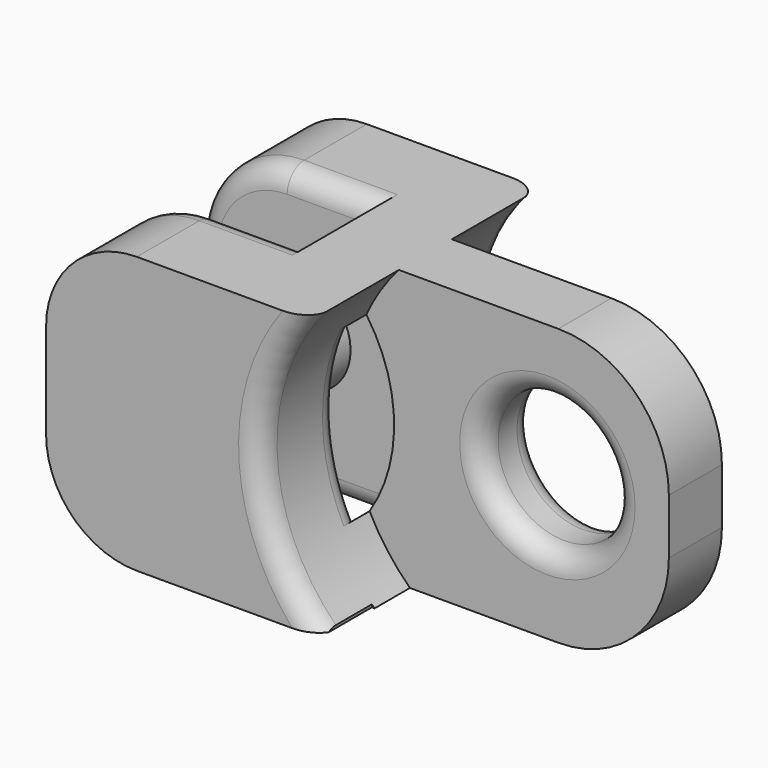
from build123d import *

# Parameters (mm, degrees)
F0_W           = 5
F0_H           = 6
F0_H_2         = 1
F0_W_2         = 13.6665210929
F0_W_3         = 3.0392452702
F0_H_3         = 8
F1_DEPTH       = 25
F2_R           = 6
F3_DEPTH       = 16.6
F4_R           = 14
F5_DEPTH       = 4
F6_R           = 4.5
F7_DEPTH       = 26
F8_R           = 18
F9_DEPTH       = 25
F10_R          = 18
F11_DEPTH      = 25
F12_R          = 10
F13_R          = 8.2083261121
F14_T1_DEPTH   = 8.5833477759
F14_T10_ANGLE  = 81.9823622478
F14_S11_R      = 14
F14_T12_DEPTH  = 16
F14_T16_ANGLE  = 81.9823622478
F14_S17_R      = 14
F14_T18_DEPTH  = 17
F14_T20_ANGLE  = 90
F14_T22_ANGLE  = 90
F14_T24_ANGLE  = 117.7013849945
F14_T26_ANGLE  = 117.7013849945
F14_T30_DEPTH  = 13.2473768354
F14_S31_R      = 14
F14_T32_DEPTH  = 8
F14_T37_DEPTH  = 8.4189497106
F14_S38_R      = 14
F14_T39_DEPTH  = 6
F14_T43_DEPTH  = 8.4189497106
F14_S44_R      = 14
F14_T45_DEPTH  = 6
F14_T49_DEPTH  = 8.4189497106
F14_S50_R      = 14
F14_T51_DEPTH  = 6
F14_T55_DEPTH  = 13.2473768354
F14_S57_R      = 14
F14_T58_DEPTH  = 8
F14_T62_DEPTH  = 8.4189497106
F14_S63_R      = 14
F14_T64_DEPTH  = 6
F14_T66_ANGLE  = 90
F14_T70_DEPTH  = 8.4189497106
F14_S71_R      = 14
F14_T72_DEPTH  = 6
F14_T76_DEPTH  = 8.4189497106
F14_S77_R      = 14
F14_T78_DEPTH  = 6
F14_T82_DEPTH  = 13.2473768354
F14_S84_R      = 14
F14_T85_DEPTH  = 8
F14_T89_DEPTH  = 8.4189497106
F14_S90_R      = 14
F14_T91_DEPTH  = 6
F14_T95_DEPTH  = 13.2473768354
F14_S97_R      = 14
F14_T98_DEPTH  = 8
F14_T102_DEPTH = 8.4189497106
F14_S103_R     = 14
F14_T104_DEPTH = 6
F14_T106_ANGLE = 90


# Not quite as in the source:
# - a fillet or chamfer that OpenCascade refuses, or shapes differently, is made with other operations: its cross-section is extruded or revolved along the edge and cut away or added


with BuildPart() as f1:
    # F0 (on Top) → F1 (new body)
    with BuildSketch(Plane.XY):
        Polygon((-5, 7), (-5, 4), (0, 4), (5, 4), (5, 7), align=None)
        Polygon((-5, -7), (5, -7), (5, -4.4536441088), (5, -4), (0, -4), (-5, -4), align=None)
        with Locations((2.5, 0)):
            Rectangle(F0_W, F0_H)
        with Locations((2.5, -3.5)):
            Rectangle(F0_W, F0_H_2)
        with Locations((2.5, 3.5)):
            Rectangle(F0_W, F0_H_2)
        Polygon((-5, -13), (-5, -7), (-5, -4), (-5, 4), (-5, 7), (-5, 13), (-29.6665210929, 13), (-29.6665210929, 4), (-13.0392452702, 4), (-10, 4), (-10, -4), (-13.0392452702, -4), (-29.6665210929, -4), (-29.6665210929, -13), align=None)
        Polygon((-5, 4), (-5, -4), (0, -4), (0, -3), (0, 3), (0, 4), align=None)
        with Locations((11.8332605464, 0)):
            Rectangle(F0_W_2, F0_H)
        with Locations((-11.5196226351, 0)):
            Rectangle(F0_W_3, F0_H_3)
    extrude(amount=F1_DEPTH)

    # F2 (on face) → F3 (cut, symmetric)
    with BuildSketch(Plane.XZ.offset(3)):
        with Locations((7.6787601748, 13.0187581394)):
            Circle(F2_R)
    extrude(amount=F3_DEPTH, both=True, mode=Mode.SUBTRACT)

    # F4 (on Front) → F5 (cut, symmetric)
    with BuildSketch(Plane.XZ):
        with Locations((-20.1836787164, 12.4924527481)):
            Circle(F4_R)
    extrude(amount=F5_DEPTH, both=True, mode=Mode.SUBTRACT)

    # F6 (on face) → F7 (join, through all)
    with BuildSketch(Plane(origin=(0, 13, 0), x_dir=(-1, 0, 0), z_dir=(0, 1, 0))):
        with Locations((20.2261688847, 12.5)):
            Circle(F6_R)
    extrude(amount=-F7_DEPTH)

    # F8 (on face) → F9 (cut)
    with BuildSketch(Plane.XZ.offset(3)):
        with Locations((7.6787601748, 13.0187581394)):
            Circle(F8_R)
        with BuildLine():
            Line((18.6665210929, 0), (5, 0))
            Line((5, 0), (5, 7.6499366742))
            ThreePointArc((5, 7.6499366742), (10.8352961679, 7.9161822679), (13.6787601748, 13.0187581394))
            ThreePointArc((13.6787601748, 13.0187581394), (10.8352961679, 18.1213340109), (5, 18.3875796047))
            Line((5, 18.3875796047), (5, 25))
            Line((5, 25), (18.6665210929, 25))
            Line((18.6665210929, 25), (18.6665210929, 0))
        make_face(mode=Mode.SUBTRACT)
    extrude(amount=F9_DEPTH, mode=Mode.SUBTRACT)

    # F10 (on face) → F11 (cut)
    with BuildSketch(Plane(origin=(0, 3, 0), x_dir=(-1, 0, 0), z_dir=(0, 1, 0))):
        with Locations((-7.6787601748, 13.0187581394)):
            Circle(F10_R)
        with BuildLine():
            Line((-5, 0), (-18.6665210929, 0))
            Line((-18.6665210929, 0), (-18.6665210929, 25))
            Line((-18.6665210929, 25), (-5, 25))
            Line((-5, 25), (-5, 18.3875796047))
            ThreePointArc((-5, 18.3875796047), (-10.8352961679, 18.1213340109), (-13.6787601748, 13.0187581394))
            ThreePointArc((-13.6787601748, 13.0187581394), (-10.8352961679, 7.9161822679), (-5, 7.6499366742))
            Line((-5, 7.6499366742), (-5, 0))
        make_face(mode=Mode.SUBTRACT)
    extrude(amount=F11_DEPTH, mode=Mode.SUBTRACT)

    # F12
    f12_edges = [f1.edges().sort_by_distance(p)[0] for p in [
        (18.666521, 0, 0),
        (18.666521, 0, 25),
    ]]
    fillet(f12_edges, radius=F12_R)

    # F13
    f13_edges = [f1.edges().sort_by_distance(p)[0] for p in [
        (-29.666521, -8.5, 0),
        (-29.666521, 8.5, 0),
        (-29.666521, 8.5, 25),
        (-29.666521, -8.5, 25),
    ]]
    fillet(f13_edges, radius=F13_R)

    # F14: fillet of radius 1.9313708499 on 16 edges, made by hand

    # F14_s2 → F14_t1 (cut)
    with BuildSketch(Plane.XY.offset(8.2083261121)):
        with BuildLine():
            ThreePointArc((-27.735150243, -4), (-29.1008356679, -4.5656854249), (-29.6665210929, -5.9313708499))
            Line((-29.6665210929, -5.9313708499), (-29.6665210929, -4))
            Line((-29.6665210929, -4), (-27.735150243, -4))
        make_face()
        with BuildLine():
            ThreePointArc((-27.735150243, 4), (-29.1008356679, 4.5656854249), (-29.6665210929, 5.9313708499))
            Line((-29.6665210929, 5.9313708499), (-29.6665210929, 4))
            Line((-29.6665210929, 4), (-27.735150243, 4))
        make_face()
    extrude(amount=F14_T1_DEPTH, mode=Mode.SUBTRACT)

    # F14_s3 → F14_t4 (revolve, cut)
    with BuildSketch(Plane.XY.offset(13.0187581394)):
        with BuildLine():
            ThreePointArc((15.6101310247, -3), (14.2444455998, -2.4343145751), (13.6787601748, -1.0686291501))
            Line((13.6787601748, -1.0686291501), (13.6787601748, -3))
            Line((13.6787601748, -3), (15.6101310247, -3))
        make_face()
    revolve(axis=Axis((7.6787601748, -3, 13.0187581394), (0, 1, 0)), mode=Mode.SUBTRACT)

    # F14_s5 → F14_t6 (revolve, cut)
    with BuildSketch(Plane.XY.offset(13.0187581394)):
        with BuildLine():
            ThreePointArc((15.6101310247, 3), (14.2444455998, 2.4343145751), (13.6787601748, 1.0686291501))
            Line((13.6787601748, 1.0686291501), (13.6787601748, 3))
            Line((13.6787601748, 3), (15.6101310247, 3))
        make_face()
    revolve(axis=Axis((7.6787601748, 3, 13.0187581394), (0, -1, 0)), mode=Mode.SUBTRACT)


with BuildPart() as f14_tool8:
    # F14_s9 → F14_t10 (revolve)
    with BuildSketch(Plane(origin=(-3.0276090133, 0, 3.3538575566), x_dir=(0, 1, 0), z_dir=(0.6700812579, 0, -0.7422877527))):
        with BuildLine():
            ThreePointArc((4, -5.5078953856), (4.5656854249, -4.1422099607), (5.9313708499, -3.5765245357))
            Line((5.9313708499, -3.5765245357), (4, -3.5765245357))
            Line((4, -3.5765245357), (4, -5.5078953856))
        make_face()
    revolve(axis=Axis((7.6787601748, 4, 13.0187581394), (0, 1, 0)), revolution_arc=F14_T10_ANGLE)

    # F14_s11 → F14_t12 (intersect, symmetric)
    with BuildSketch(Plane.XZ.offset(-5.7)):
        with Locations((-20.1836787164, 12.4924527481)):
            Circle(F14_S11_R)
    extrude(amount=F14_T12_DEPTH, both=True, mode=Mode.INTERSECT)


with BuildPart() as f1_1:
    add(f1.part)

    # F14_t7: cut F14_tool8
    add(f14_tool8.part, mode=Mode.SUBTRACT)


with BuildPart() as f14_tool14:
    # F14_s15 → F14_t16 (revolve)
    with BuildSketch(Plane(origin=(-3.0276090133, 0, 3.3538575566), x_dir=(0, 1, 0), z_dir=(0.6700812579, 0, -0.7422877527))):
        with BuildLine():
            ThreePointArc((-5.9313708499, -3.5765245357), (-4.5656854249, -4.1422099607), (-4, -5.5078953856))
            Line((-4, -5.5078953856), (-4, -3.5765245357))
            Line((-4, -3.5765245357), (-5.9313708499, -3.5765245357))
        make_face()
    revolve(axis=Axis((7.6787601748, -4, 13.0187581394), (0, 1, 0)), revolution_arc=F14_T16_ANGLE)

    # F14_s17 → F14_t18 (intersect, symmetric)
    with BuildSketch(Plane.XZ.offset(5.7)):
        with Locations((-20.1836787164, 12.4924527481)):
            Circle(F14_S17_R)
    extrude(amount=F14_T18_DEPTH, both=True, mode=Mode.INTERSECT)


with BuildPart() as f1_2:
    add(f1_1.part)

    # F14_t13: cut F14_tool14
    add(f14_tool14.part, mode=Mode.SUBTRACT)

    # F14_s19 → F14_t20 (revolve, cut)
    with BuildSketch(Plane.YZ.offset(-21.4581949808)):
        with BuildLine():
            ThreePointArc((4, 1.9313708499), (4.5656854249, 0.5656854249), (5.9313708499, 0))
            Line((5.9313708499, 0), (4, 0))
            Line((4, 0), (4, 1.9313708499))
        make_face()
    revolve(axis=Axis((-21.4581949808, 4, 8.2083261121), (0, 1, 0)), revolution_arc=F14_T20_ANGLE, mode=Mode.SUBTRACT)

    # F14_s21 → F14_t22 (revolve, cut)
    with BuildSketch(Plane.YZ.offset(-21.4581949808)):
        with BuildLine():
            ThreePointArc((-4, 1.9313708499), (-4.5656854249, 0.5656854249), (-5.9313708499, 0))
            Line((-5.9313708499, 0), (-4, 0))
            Line((-4, 0), (-4, 1.9313708499))
        make_face()
    revolve(axis=Axis((-21.4581949808, -4, 8.2083261121), (0, 1, 0)), revolution_arc=F14_T22_ANGLE, mode=Mode.SUBTRACT)

    # F14_s23 → F14_t24 (revolve, cut)
    with BuildSketch(Plane(origin=(0.2594641933, 0, -0.1462243981), x_dir=(0, 1, 0), z_dir=(0.8711795768, 0, -0.4909645049))):
        with BuildLine():
            ThreePointArc((-13, -4.8196959569), (-12.4343145751, -3.4540105319), (-11.0686291501, -2.888325107))
            Line((-11.0686291501, -2.888325107), (-13, -2.888325107))
            Line((-13, -2.888325107), (-13, -4.8196959569))
        make_face()
    revolve(axis=Axis((7.6787601748, -13, 13.0187581394), (0, 1, 0)), revolution_arc=F14_T24_ANGLE, mode=Mode.SUBTRACT)

    # F14_s25 → F14_t26 (revolve, cut)
    with BuildSketch(Plane(origin=(11.3507224474, 0, 7.3415997616), x_dir=(0, 1, 0), z_dir=(0.8396708681, 0, 0.5430956024))):
        with BuildLine():
            ThreePointArc((11.0686291501, 24.7611710656), (12.4343145751, 25.3268564905), (13, 26.6925419155))
            Line((13, 26.6925419155), (13, 24.7611710656))
            Line((13, 24.7611710656), (11.0686291501, 24.7611710656))
        make_face()
    revolve(axis=Axis((7.6787601748, 13, 13.0187581394), (0, -1, 0)), revolution_arc=F14_T26_ANGLE, mode=Mode.SUBTRACT)


with BuildPart() as f14_tool28:
    # F14_s29 → F14_t30 (new body)
    with BuildSketch(Plane.YZ.offset(-8.2108181454)):
        with BuildLine():
            ThreePointArc((-5.9313708499, 25), (-4.5656854249, 24.4343145751), (-4, 23.0686291501))
            Line((-4, 23.0686291501), (-4, 25))
            Line((-4, 25), (-5.9313708499, 25))
        make_face()
    extrude(amount=-F14_T30_DEPTH)

    # F14_s31 → F14_t32 (intersect, symmetric)
    with BuildSketch(Plane.XZ.offset(5)):
        with Locations((-20.1836787164, 12.4924527481)):
            Circle(F14_S31_R)
    extrude(amount=F14_T32_DEPTH, both=True, mode=Mode.INTERSECT)

    split(bisect_by=Plane.YZ.offset(-13.0392452702), keep=Keep.TOP)


with BuildPart() as f1_3:
    add(f1_2.part)

    # F14_t27: cut F14_tool28
    add(f14_tool28.part, mode=Mode.SUBTRACT)


with BuildPart() as f14_tool35:
    # F14_s36 → F14_t37 (new body)
    with BuildSketch(Plane.YZ.offset(-13.0392452702)):
        with BuildLine():
            ThreePointArc((-5.9313708499, 25), (-4.5656854249, 24.4343145751), (-4, 23.0686291501))
            Line((-4, 23.0686291501), (-4, 25))
            Line((-4, 25), (-5.9313708499, 25))
        make_face()
    extrude(amount=-F14_T37_DEPTH)

    # F14_s38 → F14_t39 (cut, symmetric)
    with BuildSketch(Plane.XZ.offset(5)):
        with Locations((-20.1836787164, 12.4924527481)):
            Circle(F14_S38_R)
    extrude(amount=F14_T39_DEPTH, both=True, mode=Mode.SUBTRACT)


with BuildPart() as f1_4:
    add(f1_3.part)

    # F14_t34: cut F14_tool35
    add(f14_tool35.part, mode=Mode.SUBTRACT)


with BuildPart() as f14_tool41:
    # F14_s42 → F14_t43 (new body)
    with BuildSketch(Plane.YZ.offset(-13.0392452702)):
        with BuildLine():
            ThreePointArc((-5.9313708499, 25), (-4.5656854249, 24.4343145751), (-4, 23.0686291501))
            Line((-4, 23.0686291501), (-4, 25))
            Line((-4, 25), (-5.9313708499, 25))
        make_face()
    extrude(amount=-F14_T43_DEPTH)

    # F14_s44 → F14_t45 (intersect, symmetric)
    with BuildSketch(Plane.XZ.offset(5)):
        with Locations((-20.1836787164, 12.4924527481)):
            Circle(F14_S44_R)
    extrude(amount=F14_T45_DEPTH, both=True, mode=Mode.INTERSECT)


with BuildPart() as f1_5:
    add(f1_4.part)

    # F14_t40: cut F14_tool41
    add(f14_tool41.part, mode=Mode.SUBTRACT)


with BuildPart() as f14_tool47:
    # F14_s48 → F14_t49 (new body)
    with BuildSketch(Plane.YZ.offset(-21.4581949808)):
        with BuildLine():
            ThreePointArc((5.9313708499, 25), (4.5656854249, 24.4343145751), (4, 23.0686291501))
            Line((4, 23.0686291501), (4, 25))
            Line((4, 25), (5.9313708499, 25))
        make_face()
    extrude(amount=F14_T49_DEPTH)

    # F14_s50 → F14_t51 (intersect, symmetric)
    with BuildSketch(Plane.XZ.offset(-5)):
        with Locations((-20.1836787164, 12.4924527481)):
            Circle(F14_S50_R)
    extrude(amount=F14_T51_DEPTH, both=True, mode=Mode.INTERSECT)


with BuildPart() as f1_6:
    add(f1_5.part)

    # F14_t46: cut F14_tool47
    add(f14_tool47.part, mode=Mode.SUBTRACT)


with BuildPart() as f14_tool53:
    # F14_s54 → F14_t55 (new body)
    with BuildSketch(Plane.YZ.offset(-21.4581949808)):
        with BuildLine():
            ThreePointArc((5.9313708499, 25), (4.5656854249, 24.4343145751), (4, 23.0686291501))
            Line((4, 23.0686291501), (4, 25))
            Line((4, 25), (5.9313708499, 25))
        make_face()
    extrude(amount=F14_T55_DEPTH)

    split(bisect_by=Plane.YZ.offset(-13.0392452702), keep=Keep.TOP)

    # F14_s57 → F14_t58 (intersect, symmetric)
    with BuildSketch(Plane.XZ.offset(-5)):
        with Locations((-20.1836787164, 12.4924527481)):
            Circle(F14_S57_R)
    extrude(amount=F14_T58_DEPTH, both=True, mode=Mode.INTERSECT)


with BuildPart() as f1_7:
    add(f1_6.part)

    # F14_t52: cut F14_tool53
    add(f14_tool53.part, mode=Mode.SUBTRACT)


with BuildPart() as f14_tool60:
    # F14_s61 → F14_t62 (new body)
    with BuildSketch(Plane.YZ.offset(-21.4581949808)):
        with BuildLine():
            ThreePointArc((5.9313708499, 25), (4.5656854249, 24.4343145751), (4, 23.0686291501))
            Line((4, 23.0686291501), (4, 25))
            Line((4, 25), (5.9313708499, 25))
        make_face()
    extrude(amount=F14_T62_DEPTH)

    # F14_s63 → F14_t64 (cut, symmetric)
    with BuildSketch(Plane.XZ.offset(-5)):
        with Locations((-20.1836787164, 12.4924527481)):
            Circle(F14_S63_R)
    extrude(amount=F14_T64_DEPTH, both=True, mode=Mode.SUBTRACT)


with BuildPart() as f1_8:
    add(f1_7.part)

    # F14_t59: cut F14_tool60
    add(f14_tool60.part, mode=Mode.SUBTRACT)

    # F14_s65 → F14_t66 (revolve, cut)
    with BuildSketch(Plane.YZ.offset(-21.4581949808)):
        with BuildLine():
            ThreePointArc((-5.9313708499, 25), (-4.5656854249, 24.4343145751), (-4, 23.0686291501))
            Line((-4, 23.0686291501), (-4, 25))
            Line((-4, 25), (-5.9313708499, 25))
        make_face()
    revolve(axis=Axis((-21.4581949808, -4, 16.7916738879), (0, -1, 0)), revolution_arc=F14_T66_ANGLE, mode=Mode.SUBTRACT)


with BuildPart() as f14_tool68:
    # F14_s69 → F14_t70 (new body)
    with BuildSketch(Plane.YZ.offset(-21.4581949808)):
        with BuildLine():
            ThreePointArc((-4, 1.9313708499), (-4.5656854249, 0.5656854249), (-5.9313708499, 0))
            Line((-5.9313708499, 0), (-4, 0))
            Line((-4, 0), (-4, 1.9313708499))
        make_face()
    extrude(amount=F14_T70_DEPTH)

    # F14_s71 → F14_t72 (intersect, symmetric)
    with BuildSketch(Plane.XZ.offset(5)):
        with Locations((-20.1836787164, 12.4924527481)):
            Circle(F14_S71_R)
    extrude(amount=F14_T72_DEPTH, both=True, mode=Mode.INTERSECT)


with BuildPart() as f1_9:
    add(f1_8.part)

    # F14_t67: cut F14_tool68
    add(f14_tool68.part, mode=Mode.SUBTRACT)


with BuildPart() as f14_tool74:
    # F14_s75 → F14_t76 (new body)
    with BuildSketch(Plane.YZ.offset(-21.4581949808)):
        with BuildLine():
            ThreePointArc((-4, 1.9313708499), (-4.5656854249, 0.5656854249), (-5.9313708499, 0))
            Line((-5.9313708499, 0), (-4, 0))
            Line((-4, 0), (-4, 1.9313708499))
        make_face()
    extrude(amount=F14_T76_DEPTH)

    # F14_s77 → F14_t78 (cut, symmetric)
    with BuildSketch(Plane.XZ.offset(5)):
        with Locations((-20.1836787164, 12.4924527481)):
            Circle(F14_S77_R)
    extrude(amount=F14_T78_DEPTH, both=True, mode=Mode.SUBTRACT)


with BuildPart() as f1_10:
    add(f1_9.part)

    # F14_t73: cut F14_tool74
    add(f14_tool74.part, mode=Mode.SUBTRACT)


with BuildPart() as f14_tool80:
    # F14_s81 → F14_t82 (new body)
    with BuildSketch(Plane.YZ.offset(-21.4581949808)):
        with BuildLine():
            ThreePointArc((-4, 1.9313708499), (-4.5656854249, 0.5656854249), (-5.9313708499, 0))
            Line((-5.9313708499, 0), (-4, 0))
            Line((-4, 0), (-4, 1.9313708499))
        make_face()
    extrude(amount=F14_T82_DEPTH)

    split(bisect_by=Plane.YZ.offset(-13.0392452702), keep=Keep.TOP)

    # F14_s84 → F14_t85 (intersect, symmetric)
    with BuildSketch(Plane.XZ.offset(5)):
        with Locations((-20.1836787164, 12.4924527481)):
            Circle(F14_S84_R)
    extrude(amount=F14_T85_DEPTH, both=True, mode=Mode.INTERSECT)


with BuildPart() as f1_11:
    add(f1_10.part)

    # F14_t79: cut F14_tool80
    add(f14_tool80.part, mode=Mode.SUBTRACT)


with BuildPart() as f14_tool87:
    # F14_s88 → F14_t89 (new body)
    with BuildSketch(Plane.YZ.offset(-13.0392452702)):
        with BuildLine():
            ThreePointArc((4, 1.9313708499), (4.5656854249, 0.5656854249), (5.9313708499, 0))
            Line((5.9313708499, 0), (4, 0))
            Line((4, 0), (4, 1.9313708499))
        make_face()
    extrude(amount=-F14_T89_DEPTH)

    # F14_s90 → F14_t91 (cut, symmetric)
    with BuildSketch(Plane.XZ.offset(-5)):
        with Locations((-20.1836787164, 12.4924527481)):
            Circle(F14_S90_R)
    extrude(amount=F14_T91_DEPTH, both=True, mode=Mode.SUBTRACT)


with BuildPart() as f1_12:
    add(f1_11.part)

    # F14_t86: cut F14_tool87
    add(f14_tool87.part, mode=Mode.SUBTRACT)


with BuildPart() as f14_tool93:
    # F14_s94 → F14_t95 (new body)
    with BuildSketch(Plane.YZ.offset(-8.2108181454)):
        with BuildLine():
            ThreePointArc((4, 1.9313708499), (4.5656854249, 0.5656854249), (5.9313708499, 0))
            Line((5.9313708499, 0), (4, 0))
            Line((4, 0), (4, 1.9313708499))
        make_face()
    extrude(amount=-F14_T95_DEPTH)

    split(bisect_by=Plane.YZ.offset(-13.0392452702), keep=Keep.TOP)

    # F14_s97 → F14_t98 (intersect, symmetric)
    with BuildSketch(Plane.XZ.offset(-5)):
        with Locations((-20.1836787164, 12.4924527481)):
            Circle(F14_S97_R)
    extrude(amount=F14_T98_DEPTH, both=True, mode=Mode.INTERSECT)


with BuildPart() as f1_13:
    add(f1_12.part)

    # F14_t92: cut F14_tool93
    add(f14_tool93.part, mode=Mode.SUBTRACT)


with BuildPart() as f14_tool100:
    # F14_s101 → F14_t102 (new body)
    with BuildSketch(Plane.YZ.offset(-13.0392452702)):
        with BuildLine():
            ThreePointArc((4, 1.9313708499), (4.5656854249, 0.5656854249), (5.9313708499, 0))
            Line((5.9313708499, 0), (4, 0))
            Line((4, 0), (4, 1.9313708499))
        make_face()
    extrude(amount=-F14_T102_DEPTH)

    # F14_s103 → F14_t104 (intersect, symmetric)
    with BuildSketch(Plane.XZ.offset(-5)):
        with Locations((-20.1836787164, 12.4924527481)):
            Circle(F14_S103_R)
    extrude(amount=F14_T104_DEPTH, both=True, mode=Mode.INTERSECT)


with BuildPart() as f1_14:
    add(f1_13.part)

    # F14_t99: cut F14_tool100
    add(f14_tool100.part, mode=Mode.SUBTRACT)

    # F14_s105 → F14_t106 (revolve, cut)
    with BuildSketch(Plane.YZ.offset(-21.4581949808)):
        with BuildLine():
            ThreePointArc((4, 23.0686291501), (4.5656854249, 24.4343145751), (5.9313708499, 25))
            Line((5.9313708499, 25), (4, 25))
            Line((4, 25), (4, 23.0686291501))
        make_face()
    revolve(axis=Axis((-21.4581949808, 4, 16.7916738879), (0, -1, 0)), revolution_arc=F14_T106_ANGLE, mode=Mode.SUBTRACT)


solid = f1_14.part
